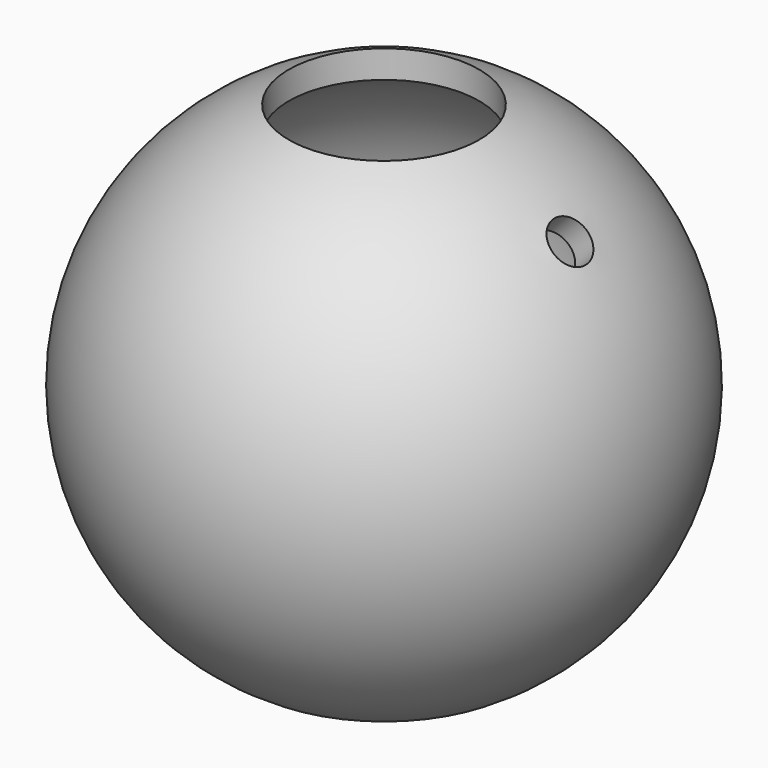
from build123d import *


with BuildPart() as f1:
    # F0 (on Right) → F1 (revolve)
    with BuildSketch(Plane.YZ):
        with BuildLine():
            Line((63.5, 3.5), (63.5, 0))
            Line((63.5, 0), (73.5, 0))
            ThreePointArc((73.5, 0), (77.3359133031, 1.5134897068), (80.9495899372, 3.5))
            Line((80.9495899372, 3.5), (63.5, 3.5))
        make_face()
        with BuildLine():
            ThreePointArc((80.9495899372, 3.5), (77.3359133031, 1.5134897068), (73.5, 0))
            Line((73.5, 0), (81.9394091831, 0))
            ThreePointArc((81.9394091831, 0), (99.4102229196, 33.9875285278), (76.5, 64.5735239147))
            Line((76.5, 64.5735239147), (76.5, 60.7901444396))
            ThreePointArc((76.5, 60.7901444396), (90.7182725546, 48.7908944847), (96.0374015748, 30.9625984252))
            ThreePointArc((96.0374015748, 30.9625984252), (92.017072223, 15.2954642562), (80.9495899372, 3.5))
        make_face()
    revolve(axis=Axis((0, 63.5, 33.5), (0, 0, -1)))

    # F3 (on line) → F4 (revolve, cut)
    with BuildSketch(Plane(origin=(0, 63.5, 0), x_dir=(-1, 0, 0), z_dir=(0, 1, 0))):
        Polygon((-27.3694280028, 58.332026428), (-21.2339044516, 52.1965028768), (-19.112584108, 54.3178232204), (-25.2481076593, 60.4533467716), align=None)
    revolve(axis=Axis((15.2781799182, 63.5, 46.2407783434), (0.7071067812, 0, 0.7071067812)), mode=Mode.SUBTRACT)


solid = f1.part
